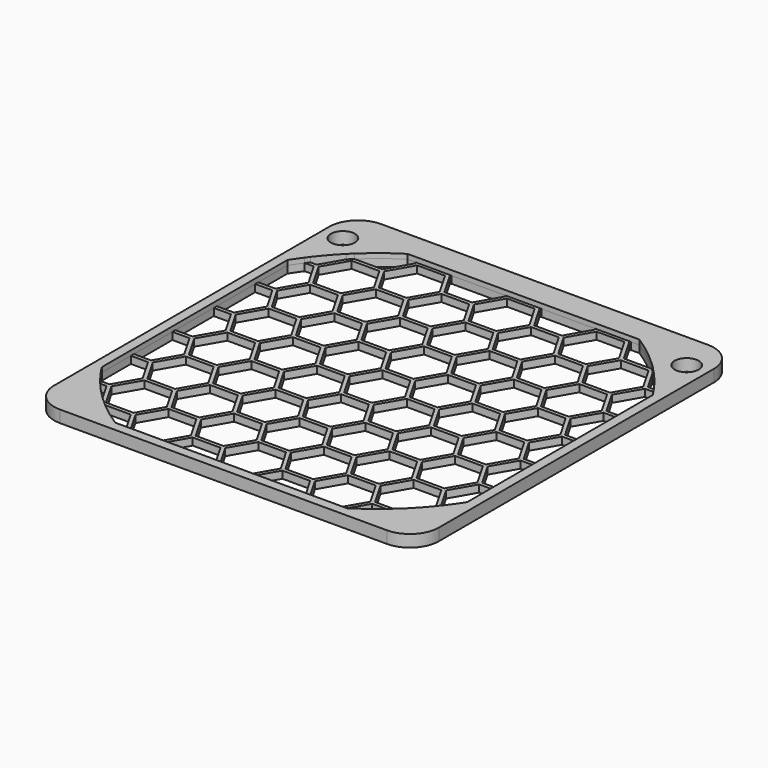
from build123d import *
from build123d import SkipClean  # not in build123d's __all__

# Parameters (mm, degrees)
F0_W     = 80
F0_H     = 83.5
F0_R     = 2.5
F1_DEPTH = 1.5
F2_W     = 80
F2_H     = 80
F2_R     = 2.5
F2_H_2   = 3.5
F3_DEPTH = 1
F4_R     = 6


with BuildPart() as f1:
    # F0 (on Top) → F1 (new body)
    with BuildSketch(Plane.XY):
        with Locations((0, 1.75)):
            Rectangle(F0_W, F0_H)
        with BuildLine():
            Line((-30.906888, -32.707251), (-25.103376, -32.707251))
            Line((-25.103376, -32.707251), (-22.216624, -37.707251))
            Line((-22.216624, -37.707251), (-22.385643, -38))
            Line((-22.385643, -38), (-24.103942, -38))
            ThreePointArc((-24.103942, -38), (-27.632429, -35.516881), (-30.906888, -32.707251))
        make_face(mode=Mode.SUBTRACT)
        with BuildLine():
            ThreePointArc((-31.857174, -31.782393), (-33.880808, -29.61572), (-35.757381, -27.3205))
            Line((-35.757381, -27.3205), (-34.433249, -27.3205))
            Line((-34.433249, -27.3205), (-31.857174, -31.782393))
        make_face(mode=Mode.SUBTRACT)
        with BuildLine():
            Line((-38, -24.103942), (-38, -16.547))
            Line((-38, -16.547), (-34.433249, -16.547))
            Line((-34.433249, -16.547), (-31.546497, -21.547))
            Line((-31.546497, -21.547), (-34.433249, -26.547))
            Line((-34.433249, -26.547), (-36.335338, -26.547))
            ThreePointArc((-36.335338, -26.547), (-37.187737, -25.339145), (-38, -24.103942))
        make_face(mode=Mode.SUBTRACT)
        Polygon((-30.876878, -21.933751), (-25.103376, -21.933751), (-22.216624, -26.933751), (-25.103376, -31.933751), (-30.876878, -31.933751), (-33.76363, -26.933751), align=None, mode=Mode.SUBTRACT)
        Polygon((-21.546751, -37.3205), (-24.433503, -32.3205), (-21.546751, -27.3205), (-15.773249, -27.3205), (-12.886497, -32.3205), (-15.773249, -37.3205), align=None, mode=Mode.SUBTRACT)
        Polygon((-12.216878, -32.707251), (-6.443376, -32.707251), (-3.556624, -37.707251), (-3.725643, -38), (-14.934611, -38), (-15.10363, -37.707251), align=None, mode=Mode.SUBTRACT)
        Polygon((-21.546751, -26.547), (-24.433503, -21.547), (-21.546751, -16.547), (-15.773249, -16.547), (-12.886497, -21.547), (-15.773249, -26.547), align=None, mode=Mode.SUBTRACT)
        Polygon((-12.216878, -21.933751), (-6.443376, -21.933751), (-3.556624, -26.933751), (-6.443376, -31.933751), (-12.216878, -31.933751), (-15.10363, -26.933751), align=None, mode=Mode.SUBTRACT)
        Polygon((-38, -15.7735), (-38, -5.7735), (-34.433249, -5.7735), (-31.546497, -10.7735), (-34.433249, -15.7735), align=None, mode=Mode.SUBTRACT)
        Polygon((-30.876878, -11.160251), (-25.103376, -11.160251), (-22.216624, -16.160251), (-25.103376, -21.160251), (-30.876878, -21.160251), (-33.76363, -16.160251), align=None, mode=Mode.SUBTRACT)
        Polygon((-38, -5), (-38, 5), (-34.433249, 5), (-31.546497, 0), (-34.433249, -5), align=None, mode=Mode.SUBTRACT)
        Polygon((-30.876878, -0.386751), (-25.103376, -0.386751), (-22.216624, -5.386751), (-25.103376, -10.386751), (-30.876878, -10.386751), (-33.76363, -5.386751), align=None, mode=Mode.SUBTRACT)
        Polygon((-21.546751, -15.7735), (-24.433503, -10.7735), (-21.546751, -5.7735), (-15.773249, -5.7735), (-12.886497, -10.7735), (-15.773249, -15.7735), align=None, mode=Mode.SUBTRACT)
        Polygon((-12.216878, -11.160251), (-6.443376, -11.160251), (-3.556624, -16.160251), (-6.443376, -21.160251), (-12.216878, -21.160251), (-15.10363, -16.160251), align=None, mode=Mode.SUBTRACT)
        Polygon((-21.546751, -5), (-24.433503, 0), (-21.546751, 5), (-15.773249, 5), (-12.886497, 0), (-15.773249, -5), align=None, mode=Mode.SUBTRACT)
        Polygon((-12.216878, -0.386751), (-6.443376, -0.386751), (-3.556624, -5.386751), (-6.443376, -10.386751), (-12.216878, -10.386751), (-15.10363, -5.386751), align=None, mode=Mode.SUBTRACT)
        Polygon((6.443122, -32.707251), (12.216624, -32.707251), (15.103376, -37.707251), (14.934357, -38), (3.725389, -38), (3.55637, -37.707251), align=None, mode=Mode.SUBTRACT)
        Polygon((-2.886751, -37.3205), (-5.773503, -32.3205), (-2.886751, -27.3205), (2.886751, -27.3205), (5.773503, -32.3205), (2.886751, -37.3205), align=None, mode=Mode.SUBTRACT)
        Polygon((15.773247, -37.3205), (12.886496, -32.3205), (15.773247, -27.3205), (21.54675, -27.3205), (24.433501, -32.3205), (21.54675, -37.3205), align=None, mode=Mode.SUBTRACT)
        Polygon((6.443122, -21.933751), (12.216624, -21.933751), (15.103376, -26.933751), (12.216624, -31.933751), (6.443122, -31.933751), (3.55637, -26.933751), align=None, mode=Mode.SUBTRACT)
        Polygon((-2.886751, -26.547), (-5.773503, -21.547), (-2.886751, -16.547), (2.886751, -16.547), (5.773503, -21.547), (2.886751, -26.547), align=None, mode=Mode.SUBTRACT)
        Polygon((15.773249, -26.547), (12.886497, -21.547), (15.773249, -16.547), (21.546751, -16.547), (24.433503, -21.547), (21.546751, -26.547), align=None, mode=Mode.SUBTRACT)
        with BuildLine():
            Line((22.21637, -37.707251), (25.103122, -32.707251))
            Line((25.103122, -32.707251), (30.906888, -32.707251))
            ThreePointArc((30.906888, -32.707251), (27.632429, -35.516881), (24.103942, -38))
            Line((24.103942, -38), (22.385389, -38))
            Line((22.385389, -38), (22.21637, -37.707251))
        make_face(mode=Mode.SUBTRACT)
        Polygon((25.103122, -21.933751), (30.876624, -21.933751), (33.763376, -26.933751), (30.876624, -31.933751), (25.103122, -31.933751), (22.21637, -26.933751), align=None, mode=Mode.SUBTRACT)
        with BuildLine():
            ThreePointArc((35.757381, -27.3205), (33.880808, -29.61572), (31.857174, -31.782393))
            Line((31.857174, -31.782393), (34.433249, -27.3205))
            Line((34.433249, -27.3205), (35.757381, -27.3205))
        make_face(mode=Mode.SUBTRACT)
        with BuildLine():
            Line((34.433249, -26.547), (31.546497, -21.547))
            Line((31.546497, -21.547), (34.433249, -16.547))
            Line((34.433249, -16.547), (38, -16.547))
            Line((38, -16.547), (38, -24.103942))
            ThreePointArc((38, -24.103942), (37.187737, -25.339145), (36.335338, -26.547))
            Line((36.335338, -26.547), (34.433249, -26.547))
        make_face(mode=Mode.SUBTRACT)
        Polygon((6.443122, -11.160251), (12.216624, -11.160251), (15.103376, -16.160251), (12.216624, -21.160251), (6.443122, -21.160251), (3.55637, -16.160251), align=None, mode=Mode.SUBTRACT)
        Polygon((-2.886751, -15.7735), (-5.773503, -10.7735), (-2.886751, -5.7735), (2.886751, -5.7735), (5.773503, -10.7735), (2.886751, -15.7735), align=None, mode=Mode.SUBTRACT)
        Polygon((15.773249, -15.7735), (12.886497, -10.7735), (15.773249, -5.7735), (21.546751, -5.7735), (24.433503, -10.7735), (21.546751, -15.7735), align=None, mode=Mode.SUBTRACT)
        Polygon((6.443122, -0.386751), (12.216624, -0.386751), (15.103376, -5.386751), (12.216624, -10.386751), (6.443122, -10.386751), (3.55637, -5.386751), align=None, mode=Mode.SUBTRACT)
        Polygon((-2.886751, -5), (-5.773503, 0), (-2.886751, 5), (2.886751, 5), (5.773503, 0), (2.886751, -5), align=None, mode=Mode.SUBTRACT)
        Polygon((15.773249, -5), (12.886497, 0), (15.773249, 5), (21.546751, 5), (24.433503, 0), (21.546751, -5), align=None, mode=Mode.SUBTRACT)
        Polygon((25.103122, -11.160251), (30.876624, -11.160251), (33.763376, -16.160251), (30.876624, -21.160251), (25.103122, -21.160251), (22.21637, -16.160251), align=None, mode=Mode.SUBTRACT)
        Polygon((34.433249, -15.7735), (31.546497, -10.7735), (34.433249, -5.7735), (38, -5.7735), (38, -15.7735), align=None, mode=Mode.SUBTRACT)
        Polygon((25.103122, -0.386751), (30.876624, -0.386751), (33.763376, -5.386751), (30.876624, -10.386751), (25.103122, -10.386751), (22.21637, -5.386751), align=None, mode=Mode.SUBTRACT)
        Polygon((34.433249, -5), (31.546497, 0), (34.433249, 5), (38, 5), (38, -5), align=None, mode=Mode.SUBTRACT)
        Polygon((-38, 5.7735), (-38, 15.7735), (-34.433249, 15.7735), (-31.546497, 10.7735), (-34.433249, 5.7735), align=None, mode=Mode.SUBTRACT)
        Polygon((-30.876878, 10.386749), (-25.103376, 10.386749), (-22.216624, 5.386749), (-25.103376, 0.386749), (-30.876878, 0.386749), (-33.76363, 5.386749), align=None, mode=Mode.SUBTRACT)
        with BuildLine():
            ThreePointArc((-38, 24.103942), (-37.187737, 25.339145), (-36.335338, 26.547))
            Line((-36.335338, 26.547), (-34.433249, 26.547))
            Line((-34.433249, 26.547), (-31.546497, 21.547))
            Line((-31.546497, 21.547), (-34.433249, 16.547))
            Line((-34.433249, 16.547), (-38, 16.547))
            Line((-38, 16.547), (-38, 24.103942))
        make_face(mode=Mode.SUBTRACT)
        Polygon((-30.876878, 21.160249), (-25.103376, 21.160249), (-22.216624, 16.160249), (-25.103376, 11.160249), (-30.876878, 11.160249), (-33.76363, 16.160249), align=None, mode=Mode.SUBTRACT)
        Polygon((-21.546751, 5.7735), (-24.433503, 10.7735), (-21.546751, 15.7735), (-15.773249, 15.7735), (-12.886497, 10.7735), (-15.773249, 5.7735), align=None, mode=Mode.SUBTRACT)
        Polygon((-12.216878, 10.386749), (-6.443376, 10.386749), (-3.556624, 5.386749), (-6.443376, 0.386749), (-12.216878, 0.386749), (-15.10363, 5.386749), align=None, mode=Mode.SUBTRACT)
        Polygon((-21.546751, 16.547), (-24.433503, 21.547), (-21.546751, 26.547), (-15.773249, 26.547), (-12.886497, 21.547), (-15.773249, 16.547), align=None, mode=Mode.SUBTRACT)
        Polygon((-12.216878, 21.160249), (-6.443376, 21.160249), (-3.556624, 16.160249), (-6.443376, 11.160249), (-12.216878, 11.160249), (-15.10363, 16.160249), align=None, mode=Mode.SUBTRACT)
        with BuildLine():
            ThreePointArc((-35.757381, 27.3205), (-33.880808, 29.61572), (-31.857174, 31.782393))
            Line((-31.857174, 31.782393), (-34.433249, 27.3205))
            Line((-34.433249, 27.3205), (-35.757381, 27.3205))
        make_face(mode=Mode.SUBTRACT)
        Polygon((-30.876878, 31.933749), (-25.103376, 31.933749), (-22.216624, 26.933749), (-25.103376, 21.933749), (-30.876878, 21.933749), (-33.76363, 26.933749), align=None, mode=Mode.SUBTRACT)
        with Locations((-35.75, 35.75)):
            Circle(F0_R, mode=Mode.SUBTRACT)
        with BuildLine():
            Line((-24.103942, 38), (-22.385644, 38))
            Line((-22.385644, 38), (-22.216624, 37.707249))
            Line((-22.216624, 37.707249), (-25.103376, 32.707249))
            Line((-25.103376, 32.707249), (-30.906891, 32.707249))
            ThreePointArc((-30.906891, 32.707249), (-27.632431, 35.51688), (-24.103942, 38))
        make_face(mode=Mode.SUBTRACT)
        Polygon((-21.546751, 27.3205), (-24.433503, 32.3205), (-21.546751, 37.3205), (-15.773249, 37.3205), (-12.886497, 32.3205), (-15.773249, 27.3205), align=None, mode=Mode.SUBTRACT)
        Polygon((-12.216878, 31.933749), (-6.443376, 31.933749), (-3.556624, 26.933749), (-6.443376, 21.933749), (-12.216878, 21.933749), (-15.10363, 26.933749), align=None, mode=Mode.SUBTRACT)
        Polygon((-14.934609, 38), (-3.725644, 38), (-3.556624, 37.707249), (-6.443376, 32.707249), (-12.216878, 32.707249), (-15.10363, 37.707249), align=None, mode=Mode.SUBTRACT)
        Polygon((6.443122, 10.386749), (12.216624, 10.386749), (15.103376, 5.386749), (12.216624, 0.386749), (6.443122, 0.386749), (3.55637, 5.386749), align=None, mode=Mode.SUBTRACT)
        Polygon((-2.886751, 5.7735), (-5.773503, 10.7735), (-2.886751, 15.7735), (2.886751, 15.7735), (5.773503, 10.7735), (2.886751, 5.7735), align=None, mode=Mode.SUBTRACT)
        Polygon((15.773249, 5.7735), (12.886497, 10.7735), (15.773249, 15.7735), (21.546751, 15.7735), (24.433503, 10.7735), (21.546751, 5.7735), align=None, mode=Mode.SUBTRACT)
        Polygon((6.443122, 21.160249), (12.216624, 21.160249), (15.103376, 16.160249), (12.216624, 11.160249), (6.443122, 11.160249), (3.55637, 16.160249), align=None, mode=Mode.SUBTRACT)
        Polygon((-2.886751, 16.547), (-5.773503, 21.547), (-2.886751, 26.547), (2.886751, 26.547), (5.773503, 21.547), (2.886751, 16.547), align=None, mode=Mode.SUBTRACT)
        Polygon((15.773249, 16.547), (12.886497, 21.547), (15.773249, 26.547), (21.546751, 26.547), (24.433503, 21.547), (21.546751, 16.547), align=None, mode=Mode.SUBTRACT)
        Polygon((25.103122, 10.386749), (30.876624, 10.386749), (33.763376, 5.386749), (30.876624, 0.386749), (25.103122, 0.386749), (22.21637, 5.386749), align=None, mode=Mode.SUBTRACT)
        Polygon((34.433249, 5.7735), (31.546497, 10.7735), (34.433249, 15.7735), (38, 15.7735), (38, 5.7735), align=None, mode=Mode.SUBTRACT)
        Polygon((25.103122, 21.160249), (30.876624, 21.160249), (33.763376, 16.160249), (30.876624, 11.160249), (25.103122, 11.160249), (22.21637, 16.160249), align=None, mode=Mode.SUBTRACT)
        with BuildLine():
            Line((34.433249, 16.547), (31.546497, 21.547))
            Line((31.546497, 21.547), (34.433249, 26.547))
            Line((34.433249, 26.547), (36.335338, 26.547))
            ThreePointArc((36.335338, 26.547), (37.187737, 25.339144), (38, 24.103942))
            Line((38, 24.103942), (38, 16.547))
            Line((38, 16.547), (34.433249, 16.547))
        make_face(mode=Mode.SUBTRACT)
        Polygon((6.443122, 31.933749), (12.216624, 31.933749), (15.103376, 26.933749), (12.216624, 21.933749), (6.443122, 21.933749), (3.55637, 26.933749), align=None, mode=Mode.SUBTRACT)
        Polygon((-2.886751, 27.3205), (-5.773503, 32.3205), (-2.886751, 37.3205), (2.886751, 37.3205), (5.773503, 32.3205), (2.886751, 27.3205), align=None, mode=Mode.SUBTRACT)
        Polygon((15.773249, 27.3205), (12.886497, 32.3205), (15.773249, 37.3205), (21.546751, 37.3205), (24.433503, 32.3205), (21.546751, 27.3205), align=None, mode=Mode.SUBTRACT)
        Polygon((3.725391, 38), (14.934356, 38), (15.103376, 37.707249), (12.216624, 32.707249), (6.443122, 32.707249), (3.55637, 37.707249), align=None, mode=Mode.SUBTRACT)
        Polygon((25.103122, 31.933749), (30.876624, 31.933749), (33.763376, 26.933749), (30.876624, 21.933749), (25.103122, 21.933749), (22.21637, 26.933749), align=None, mode=Mode.SUBTRACT)
        with BuildLine():
            Line((35.757381, 27.3205), (34.433249, 27.3205))
            Line((34.433249, 27.3205), (31.857174, 31.782393))
            ThreePointArc((31.857174, 31.782393), (33.880808, 29.61572), (35.757381, 27.3205))
        make_face(mode=Mode.SUBTRACT)
        with BuildLine():
            Line((30.887304, 32.725746), (30.876624, 32.707249))
            Line((30.876624, 32.707249), (25.103122, 32.707249))
            Line((25.103122, 32.707249), (22.21637, 37.707249))
            Line((22.21637, 37.707249), (22.385391, 38))
            Line((22.385391, 38), (24.103942, 38))
            ThreePointArc((24.103942, 38), (27.621798, 35.52515), (30.887304, 32.725746))
        make_face(mode=Mode.SUBTRACT)
        with Locations((35.75, 35.75)):
            Circle(F0_R, mode=Mode.SUBTRACT)
    extrude(amount=F1_DEPTH)

    # F2 (on face) → F3 (join)
    with BuildSketch(Plane.XY.offset(1.5)):
        Rectangle(F2_W, F2_H)
        with BuildLine():
            Line((37.999999, -16.547), (37.999999, -24.103944))
            ThreePointArc((37.999999, -24.103944), (37.187736, -25.339145), (36.335338, -26.547))
            ThreePointArc((36.335338, -26.547), (36.048434, -26.9353), (35.757381, -27.3205))
            ThreePointArc((35.757381, -27.3205), (33.880808, -29.61572), (31.857174, -31.782393))
            ThreePointArc((31.857174, -31.782393), (31.385438, -32.248323), (30.906888, -32.707251))
            ThreePointArc((30.906888, -32.707251), (27.63243, -35.516881), (24.103944, -37.999999))
            Line((24.103944, -37.999999), (22.385389, -37.999999))
            Line((22.385389, -37.999999), (14.934357, -37.999999))
            Line((14.934357, -37.999999), (3.725389, -37.999999))
            Line((3.725389, -37.999999), (-3.725643, -37.999999))
            Line((-3.725643, -37.999999), (-14.934611, -37.999999))
            Line((-14.934611, -37.999999), (-22.385643, -37.999999))
            Line((-22.385643, -37.999999), (-24.103944, -37.999999))
            ThreePointArc((-24.103944, -37.999999), (-27.63243, -35.516881), (-30.906888, -32.707251))
            ThreePointArc((-30.906888, -32.707251), (-31.385438, -32.248323), (-31.857174, -31.782393))
            ThreePointArc((-31.857174, -31.782393), (-33.880808, -29.61572), (-35.757381, -27.3205))
            ThreePointArc((-35.757381, -27.3205), (-36.048434, -26.9353), (-36.335338, -26.547))
            ThreePointArc((-36.335338, -26.547), (-37.187736, -25.339145), (-37.999999, -24.103944))
            Line((-37.999999, -24.103944), (-37.999999, -16.547))
            Line((-37.999999, -16.547), (-37.999999, -15.7735))
            Line((-37.999999, -15.7735), (-37.999999, -5.7735))
            Line((-37.999999, -5.7735), (-37.999999, -5))
            Line((-37.999999, -5), (-37.999999, 5))
            Line((-37.999999, 5), (-37.999999, 5.7735))
            Line((-37.999999, 5.7735), (-37.999999, 15.7735))
            Line((-37.999999, 15.7735), (-37.999999, 16.547))
            Line((-37.999999, 16.547), (-37.999999, 24.103944))
            ThreePointArc((-37.999999, 24.103944), (-37.187736, 25.339145), (-36.335338, 26.547))
            ThreePointArc((-36.335338, 26.547), (-36.048434, 26.9353), (-35.757381, 27.3205))
            ThreePointArc((-35.757381, 27.3205), (-33.880808, 29.61572), (-31.857174, 31.782393))
            ThreePointArc((-31.857174, 31.782393), (-31.385439, 32.248321), (-30.906891, 32.707249))
            ThreePointArc((-30.906891, 32.707249), (-27.632432, 35.516879), (-24.103944, 37.999999))
            Line((-24.103944, 37.999999), (-22.385644, 37.999999))
            Line((-22.385644, 37.999999), (-14.934609, 37.999999))
            Line((-14.934609, 37.999999), (-3.725644, 37.999999))
            Line((-3.725644, 37.999999), (3.725391, 37.999999))
            Line((3.725391, 37.999999), (14.934356, 37.999999))
            Line((14.934356, 37.999999), (22.385391, 37.999999))
            Line((22.385391, 37.999999), (24.103944, 37.999999))
            ThreePointArc((24.103944, 37.999999), (27.621799, 35.525149), (30.887304, 32.725746))
            ThreePointArc((30.887304, 32.725746), (31.375784, 32.257715), (31.857174, 31.782393))
            ThreePointArc((31.857174, 31.782393), (33.880808, 29.61572), (35.757381, 27.3205))
            ThreePointArc((35.757381, 27.3205), (36.048434, 26.9353), (36.335338, 26.547))
            ThreePointArc((36.335338, 26.547), (37.187736, 25.339145), (37.999999, 24.103944))
            Line((37.999999, 24.103944), (37.999999, 16.547))
            Line((37.999999, 16.547), (37.999999, 15.7735))
            Line((37.999999, 15.7735), (37.999999, 5.7735))
            Line((37.999999, 5.7735), (37.999999, 5))
            Line((37.999999, 5), (37.999999, -5))
            Line((37.999999, -5), (37.999999, -5.7735))
            Line((37.999999, -5.7735), (37.999999, -15.7735))
            Line((37.999999, -15.7735), (37.999999, -16.547))
        make_face(mode=Mode.SUBTRACT)
        with Locations((-35.75, 35.75)):
            Circle(F2_R, mode=Mode.SUBTRACT)
        with Locations((35.75, 35.75)):
            Circle(F2_R, mode=Mode.SUBTRACT)
        with Locations((0, 41.75)):
            Rectangle(F2_W, F2_H_2)
    with SkipClean():  # cleaning this boolean's faces spoils the solid; the shape is the same uncleaned
        extrude(amount=F3_DEPTH)

    # F4
    f4_edges = [f1.edges().sort_by_distance(p)[0] for p in [
        (-40, 43.5, 0.75),
        (-40, 43.5, 2),
        (-40, -40, 0.75),
        (-40, -40, 2),
        (40, -40, 0.75),
        (40, -40, 2),
        (40, 43.5, 0.75),
        (40, 43.5, 2),
    ]]
    fillet(f4_edges, radius=F4_R)


solid = f1.part
